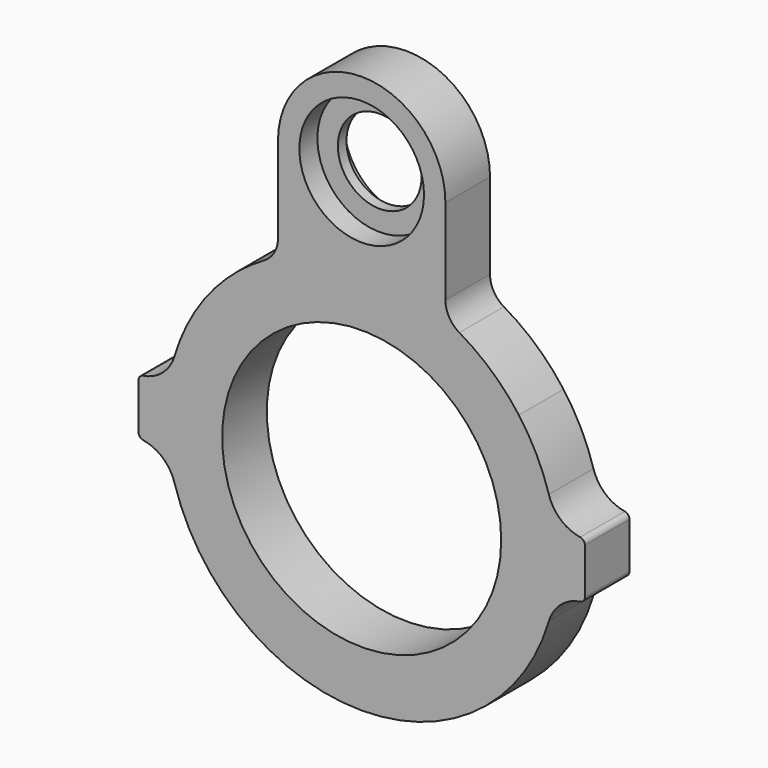
from build123d import *

# Parameters (mm, degrees)
F0_R        = 31.75
F0_R_2      = 9.525
F1_DEPTH    = 12.7
F2_T1_DEPTH = 12.7
F3_R        = 1.27
F4_R        = 14.1859
F4_R_2      = 9.525
F5_DEPTH    = 5.1308
F6_R        = 14.1859
F6_R_2      = 9.525
F7_DEPTH    = 5.1308


# Not quite as in the source:
# - a fillet or chamfer that OpenCascade refuses, or shapes differently, is made with other operations: its cross-section is extruded or revolved along the edge and cut away or added


with BuildPart() as f1:
    # F0 (on Front) → F1 (new body)
    with BuildSketch(Plane.XZ):
        with BuildLine():
            Line((19.05, 12.2440905122), (19.05, 31.75))
            ThreePointArc((19.05, 31.75), (0, 50.8), (-19.05, 31.75))
            Line((-19.05, 31.75), (-19.05, 12.2440905122))
            ThreePointArc((-19.05, 12.2440905122), (-19.900738686, 9.0690905122), (-22.225, 6.7448291982))
            ThreePointArc((-22.225, 6.7448291982), (-29.6221228011, 1.3910974586), (-35.7691769709, -5.3612054307))
            ThreePointArc((-35.7691769709, -5.3612054307), (-41.1209561154, -14.8719234463), (-43.9940905122, -25.4))
            Line((-43.9940905122, -25.4), (-50.8, -25.4))
            Line((-50.8, -25.4), (-50.8, -38.1))
            Line((-50.8, -38.1), (-43.9940905122, -38.1))
            ThreePointArc((-43.9940905122, -38.1), (0, -76.2), (43.9940905122, -38.1))
            Line((43.9940905122, -38.1), (50.8, -38.1))
            Line((50.8, -38.1), (50.8, -25.4))
            Line((50.8, -25.4), (43.9940905122, -25.4))
            ThreePointArc((43.9940905122, -25.4), (41.1209561154, -14.8719234463), (35.7691769709, -5.3612054307))
            ThreePointArc((35.7691769709, -5.3612054307), (29.6221228011, 1.3910974586), (22.225, 6.7448291982))
            ThreePointArc((22.225, 6.7448291982), (19.900738686, 9.0690905122), (19.05, 12.2440905122))
        make_face()
        with Locations((0, -31.75)):
            Circle(F0_R, mode=Mode.SUBTRACT)
        with Locations((0, 31.75)):
            Circle(F0_R_2, mode=Mode.SUBTRACT)
    extrude(amount=F1_DEPTH)

    # F2: fillet of radius 8.89 on 4 edges, made by hand

    # F2_s2 → F2_t1 (join)
    with BuildSketch(Plane.XZ):
        with BuildLine():
            ThreePointArc((-50.8, -25.4), (-45.6782912458, -23.5470098171), (-42.5985100968, -19.0547474412))
            ThreePointArc((-42.5985100968, -19.0547474412), (-43.4123850712, -22.2018419352), (-43.9940905122, -25.4))
            Line((-43.9940905122, -25.4), (-50.8, -25.4))
        make_face()
        with BuildLine():
            ThreePointArc((50.8, -25.4), (45.6782912458, -23.5470098171), (42.5985100968, -19.0547474412))
            ThreePointArc((42.5985100968, -19.0547474412), (43.4123850712, -22.2018419352), (43.9940905122, -25.4))
            Line((43.9940905122, -25.4), (50.8, -25.4))
        make_face()
        with BuildLine():
            ThreePointArc((-42.5985100968, -44.4452525588), (-45.6782912458, -39.9529901829), (-50.8, -38.1))
            Line((-50.8, -38.1), (-43.9940905122, -38.1))
            ThreePointArc((-43.9940905122, -38.1), (-43.4123850712, -41.2981580648), (-42.5985100968, -44.4452525588))
        make_face()
        with BuildLine():
            ThreePointArc((50.8, -38.1), (45.6782912458, -39.9529901829), (42.5985100968, -44.4452525588))
            ThreePointArc((42.5985100968, -44.4452525588), (43.4123850712, -41.2981580648), (43.9940905122, -38.1))
            Line((43.9940905122, -38.1), (50.8, -38.1))
        make_face()
    extrude(amount=F2_T1_DEPTH)

    # F3
    f3_edges = [f1.edges().sort_by_distance(p)[0] for p in [
        (-50.8, -6.35, -25.4),
        (-50.8, -6.35, -38.1),
        (50.8, -6.35, -25.4),
        (50.8, -6.35, -38.1),
    ]]
    fillet(f3_edges, radius=F3_R)

    # F4 (on face) → F5 (cut)
    with BuildSketch(Plane.XZ.offset(12.7)):
        with Locations((0, 31.75)):
            Circle(F4_R)
        with Locations((0, 31.75)):
            Circle(F4_R_2, mode=Mode.SUBTRACT)
    extrude(amount=-F5_DEPTH, mode=Mode.SUBTRACT)

    # F6 (on face) → F7 (cut)
    with BuildSketch(Plane(origin=(0, 0, 0), x_dir=(-1, 0, 0), z_dir=(0, 1, 0))):
        with Locations((0, 31.75)):
            Circle(F6_R)
        with Locations((0, 31.75)):
            Circle(F6_R_2, mode=Mode.SUBTRACT)
    extrude(amount=-F7_DEPTH, mode=Mode.SUBTRACT)


solid = f1.part
